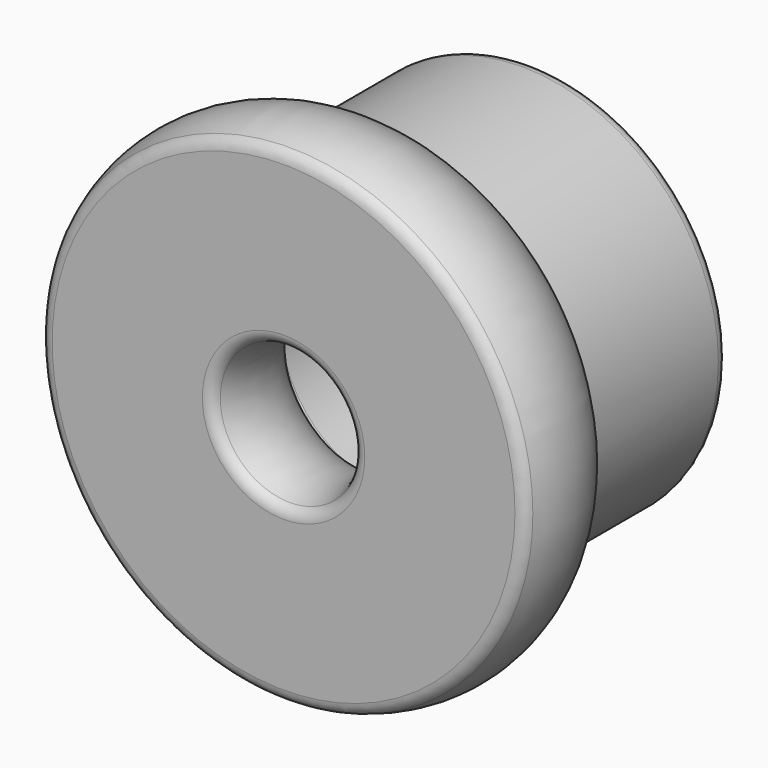
from build123d import *

# Parameters (mm, degrees)
F2_R = 5.08
F3_R = 5.08


# Not quite as in the source:
# - a fillet or chamfer that OpenCascade refuses, or shapes differently, is made with other operations: its cross-section is extruded or revolved along the edge and cut away or added


with BuildPart() as f1:
    # F0 (on Top) → F1 (revolve)
    with BuildSketch(Plane.XY):
        Polygon((15.8496014774, 59.5883987844), (-18.2879995555, 59.5883987844), (-18.2879995555, -12.9540003836), (-17.6547473952, -12.9540003836), (15.8496014774, -12.9540003836), (15.8496014774, -12.0559275107), align=None)
        with BuildLine():
            ThreePointArc((33.0465635914, -64.1603991389), (35.7271287753, -34.3855398181), (15.8496014774, -12.0559275107))
            Line((15.8496014774, -12.0559275107), (15.8496014774, -12.9540003836))
            Line((15.8496014774, -12.9540003836), (-17.6547473952, -12.9540003836))
            ThreePointArc((-17.6547473952, -12.9540003836), (-36.0302588433, -35.3470835296), (-33.0465635914, -64.1603991389))
            Line((-33.0465635914, -64.1603991389), (33.0465635914, -64.1603991389))
        make_face()
    revolve(axis=Axis((-62.1792003512, -0.6096027792, 0), (0, -1, 0)))

    # F2
    f2_edges = [f1.edges().sort_by_distance(p)[0] for p in [
        (-157.404964, -64.160399, 0),
        (-140.208002, 59.588399, 0),
    ]]
    fillet(f2_edges, radius=F2_R)

    # F3
    f3_edges = [f1.edges().sort_by_distance(p)[0] for p in [
        (-140.208002, -12.055928, 0),
    ]]
    fillet(f3_edges, radius=F3_R)

    # F4: fillet of radius 5.08 on 3 edges, made by hand

    # F4_s1 → F4_t2 (revolve, cut)
    with BuildSketch(Plane.XY):
        with BuildLine():
            ThreePointArc((-13.2079995555, 59.5883987844), (-16.8001020039, 58.1005012328), (-18.2879995555, 54.5083987844))
            Line((-18.2879995555, 54.5083987844), (-18.2879995555, 59.5883987844))
            Line((-18.2879995555, 59.5883987844), (-13.2079995555, 59.5883987844))
        make_face()
    revolve(axis=Axis((-62.1792003512, 59.5883987844, 0), (0, -1, 0)), mode=Mode.SUBTRACT)

    # F4_s3 → F4_t4 (revolve, cut)
    with BuildSketch(Plane.XY):
        with BuildLine():
            ThreePointArc((-18.2879995555, -10.4978176442), (-18.1271396747, -11.7660686), (-17.6547473952, -12.9540003836))
            Line((-17.6547473952, -12.9540003836), (-18.2879995555, -12.9540003836))
            Line((-18.2879995555, -12.9540003836), (-18.2879995555, -10.4978176442))
        make_face()
    revolve(axis=Axis((-62.1792003512, -12.9540003836, 0), (0, -1, 0)), mode=Mode.SUBTRACT)

    # F4_s5 → F4_t6 (revolve, cut)
    with BuildSketch(Plane.XY):
        with BuildLine():
            ThreePointArc((-29.8753679594, -64.1603991389), (-32.6659019153, -63.3253161277), (-34.5389840999, -61.0946197064))
            ThreePointArc((-34.5389840999, -61.0946197064), (-33.8275230407, -62.6444253203), (-33.0465635914, -64.1603991389))
            Line((-33.0465635914, -64.1603991389), (-29.8753679594, -64.1603991389))
        make_face()
    revolve(axis=Axis((-62.1792003512, -64.1603991389, 0), (0, -1, 0)), mode=Mode.SUBTRACT)


solid = f1.part
